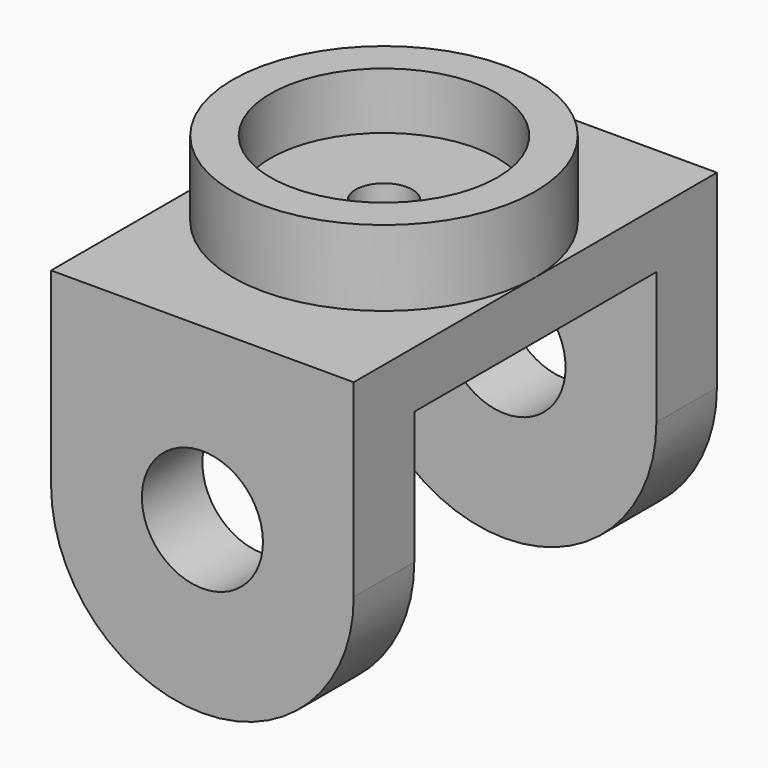
from build123d import *

# Parameters (mm, degrees)
F0_W          = 80
F0_H          = 90
F1_DEPTH      = 60
F1_DEPTH_BACK = 60
F2_R          = 39.99999
F3_R          = 16
F4_DEPTH      = 120.001
F5_W          = 80
F5_H          = 64.99999
F5_H_2        = 35.00001
F6_DEPTH      = 80.001
F7_R          = 7.5
F8_DEPTH      = 90.001
F7_R_2        = 30
F9_DEPTH      = 5
F10_DEPTH     = 20


# Not quite as in the source:
# - a fillet or chamfer is up to 0.001 mm smaller than in the source, because OpenCascade refuses the exact size


with BuildPart() as f1:
    # F0 (on Front) → F1 (new body, two sides)
    with BuildSketch(Plane.XZ) as f1_sk:
        Rectangle(F0_W, F0_H)
    extrude(amount=F1_DEPTH)
    extrude(f1_sk.sketch, amount=-F1_DEPTH_BACK)

    # F2 (radius 40 in the source; OpenCascade refuses exactly that, so slightly less here)
    f2_edges = [f1.edges().sort_by_distance(p)[0] for p in [
        (40, 0, -45),
        (-40, 0, -45),
    ]]
    fillet(f2_edges, radius=F2_R)

    # F3 (on face) → F4 (cut, through all)
    with BuildSketch(Plane.XZ.offset(60)):
        Circle(F3_R)
    extrude(amount=-F4_DEPTH, mode=Mode.SUBTRACT)

    # F5 (on face) → F6 (cut, through all)
    with BuildSketch(Plane(origin=(-40, 0, 0), x_dir=(0, -1, 0), z_dir=(-1, 0, 0))):
        with Locations((0, -37.500005)):
            Rectangle(F5_W, F5_H)
        with Locations((0, 12.499995)):
            Rectangle(F5_W, F5_H_2)
    extrude(amount=-F6_DEPTH, mode=Mode.SUBTRACT)

    # F7 (on face) → F8 (cut, through all)
    with BuildSketch(Plane.XY.offset(45)):
        Circle(F7_R)
    extrude(amount=-F8_DEPTH, mode=Mode.SUBTRACT)

    # F7 (on face) → F9 (join)
    with BuildSketch(Plane.XY.offset(45)):
        Circle(F7_R_2)
        Circle(F7_R, mode=Mode.SUBTRACT)
    extrude(amount=F9_DEPTH)

    # F7 (on face) → F10 (join)
    with BuildSketch(Plane.XY.offset(45)):
        with BuildLine():
            ThreePointArc((-40, 0), (0, -40), (40, 0))
            ThreePointArc((40, 0), (0, 40), (-40, 0))
        make_face()
        Circle(F7_R_2, mode=Mode.SUBTRACT)
    extrude(amount=F10_DEPTH)


solid = f1.part
